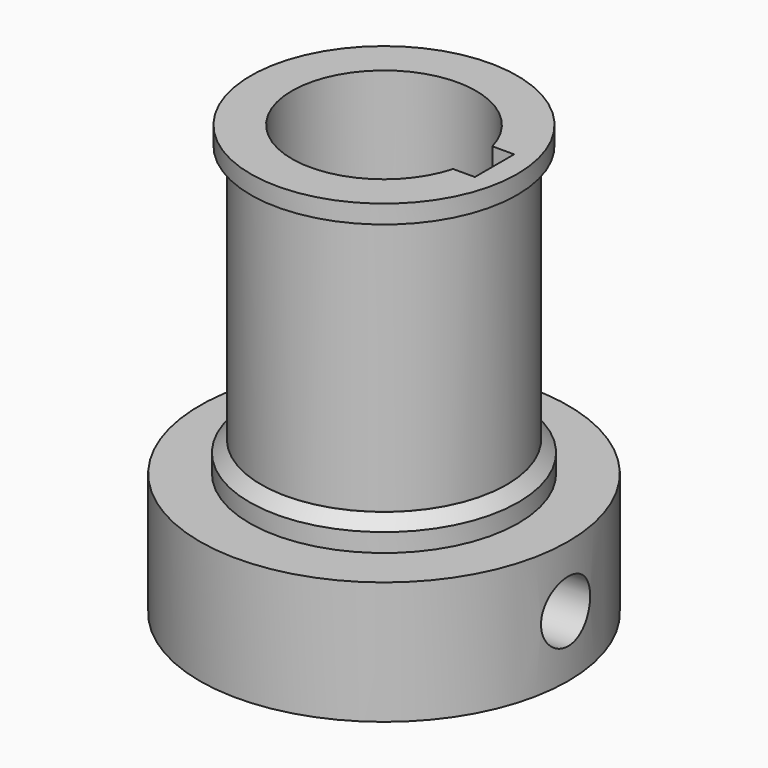
from build123d import *

# Parameters (mm, degrees)
F0_R         = 30
F1_DEPTH     = 20
F2_R         = 21.9
F3_DEPTH     = 5
F4_R         = 20
F5_DEPTH     = 42
F6_R         = 21.7
F6_R_2       = 20
F7_DEPTH     = 3
F9_D         = 10
F9_DEPTH     = 80
F9_TIP       = 3.0043030951
F11_D        = 10
F11_DEPTH    = 50
F11_TIP      = 3.0043030951
F12_S5_R     = 20
F12_T6_DEPTH = 32


# Not quite as in the source:
# - a fillet or chamfer that OpenCascade refuses, or shapes differently, is made with other operations: its cross-section is extruded or revolved along the edge and cut away or added


with BuildPart() as f1:
    # F0 (on Top) → F1 (new body)
    with BuildSketch(Plane.XY):
        Circle(F0_R)
        with BuildLine():
            ThreePointArc((14.4568322948, -4), (-15, 0), (14.4568322948, 4))
            Line((14.4568322948, 4), (18, 4))
            Line((18, 4), (18, 0))
            Line((18, 0), (18, -4))
            Line((18, -4), (14.4568322948, -4))
        make_face(mode=Mode.SUBTRACT)
    extrude(amount=F1_DEPTH)

    # F2 (on face) → F3 (join)
    with BuildSketch(Plane.XY.offset(20)):
        Circle(F2_R)
        with BuildLine():
            ThreePointArc((14.4568322948, -4), (-15, 0), (14.4568322948, 4))
            Line((14.4568322948, 4), (18, 4))
            Line((18, 4), (18, -4))
            Line((18, -4), (14.4568322948, -4))
        make_face(mode=Mode.SUBTRACT)
    extrude(amount=F3_DEPTH)

    # F4 (on face) → F5 (join)
    with BuildSketch(Plane.XY.offset(25)):
        Circle(F4_R)
        with BuildLine():
            ThreePointArc((14.4568322948, -4), (-15, 0), (14.4568322948, 4))
            Line((14.4568322948, 4), (18, 4))
            Line((18, 4), (18, -4))
            Line((18, -4), (14.4568322948, -4))
        make_face(mode=Mode.SUBTRACT)
    extrude(amount=F5_DEPTH)

    # F6 (on face) → F7 (join)
    with BuildSketch(Plane.XY.offset(67)):
        Circle(F6_R)
        Circle(F6_R_2, mode=Mode.SUBTRACT)
        Circle(F6_R_2)
        with BuildLine():
            ThreePointArc((14.4568322948, -4), (-15, 0), (14.4568322948, 4))
            Line((14.4568322948, 4), (18, 4))
            Line((18, 4), (18, -4))
            Line((18, -4), (14.4568322948, -4))
        make_face(mode=Mode.SUBTRACT)
    extrude(amount=F7_DEPTH)

    # F9 (one way)
    with BuildSketch(Plane(origin=(0, 0, 0), x_dir=(0, 1, 0), z_dir=(-1, 0, 0))):
        with Locations((0, -10)):
            Circle(F9_D / 2)
    extrude(amount=-F9_DEPTH, mode=Mode.SUBTRACT)
    with Locations(Plane(origin=(0, 0, 0), x_dir=(0, 1, 0), z_dir=(-1, 0, 0))):
        with Locations((0, -10)):
            with Locations((0, 0, -(F9_DEPTH + F9_TIP / 2))):  # 118° drill point
                Cone(0, F9_D / 2, F9_TIP, mode=Mode.SUBTRACT)

    # F11 (one way)
    with BuildSketch(Plane.XZ):
        with Locations((0, 10)):
            Circle(F11_D / 2)
    extrude(amount=-F11_DEPTH, mode=Mode.SUBTRACT)
    with Locations(Plane.XZ):
        with Locations((0, 10)):
            with Locations((0, 0, -(F11_DEPTH + F11_TIP / 2))):  # 118° drill point
                Cone(0, F11_D / 2, F11_TIP, mode=Mode.SUBTRACT)

    # F12: chamfer of 2 on 1 edges, made by hand


with BuildPart() as f12_tool2:
    # F12_s3 → F12_t4 (revolve)
    with BuildSketch(Plane.XZ):
        Polygon((21.9, 23), (19.9, 25), (21.9, 25), align=None)
    revolve(axis=Axis((0, 0, 25), (0, 0, 1)))

    # F12_s5 → F12_t6 (cut, symmetric)
    with BuildSketch(Plane.XY.offset(24)):
        Circle(F12_S5_R)
    extrude(amount=F12_T6_DEPTH, both=True, mode=Mode.SUBTRACT)


with BuildPart() as f1_1:
    add(f1.part)

    # F12_t1: cut F12_tool2
    add(f12_tool2.part, mode=Mode.SUBTRACT)


solid = f1_1.part
